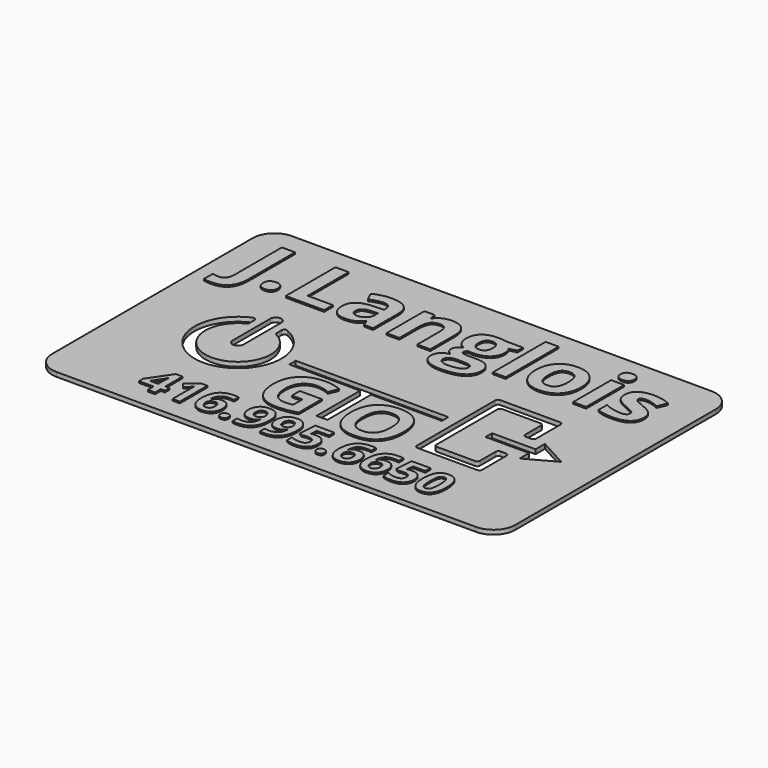
from build123d import *

# Parameters (mm, degrees)
F1_DEPTH       = 0.8
F3_DEPTH       = 0.801
F4_TEXT_SIZE   = 7.0678230889
F5_DEPTH       = 0.3
F6_TEXT_SIZE   = 15.9617374922
F6_TEXT_SIZE_2 = 8.8388333097
F6_TEXT_SIZE_3 = 14.3189125487
F7_DEPTH       = 0.3


# Not quite as in the source:
# - Text() gives the source's letters only with a copy of the font that has no kerning and outlines rounded to 1/6400 em; it was checked with that copy


with BuildPart() as f1:
    # F0 (on Top) → F1 (new body)
    with BuildSketch(Plane.XY):
        with BuildLine():
            ThreePointArc((42.4102088809, 23.1660448015), (41.2386360056, 25.9944719262), (38.4102088809, 27.1660448015))
            Line((38.4102088809, 27.1660448015), (-38.5897911191, 27.1660448015))
            ThreePointArc((-38.5897911191, 27.1660448015), (-41.4182182438, 25.9944719262), (-42.5897911191, 23.1660448015))
            Line((-42.5897911191, 23.1660448015), (-42.5897911191, -22.8339551985))
            ThreePointArc((-42.5897911191, -22.8339551985), (-41.4182182438, -25.6623823233), (-38.5897911191, -26.8339551985))
            Line((-38.5897911191, -26.8339551985), (38.4102088809, -26.8339551985))
            ThreePointArc((38.4102088809, -26.8339551985), (41.2386360056, -25.6623823233), (42.4102088809, -22.8339551985))
            Line((42.4102088809, -22.8339551985), (42.4102088809, 23.1660448015))
        make_face()
    extrude(amount=F1_DEPTH)

    # F2 (on face) → F3 (cut, through all)
    with BuildSketch(Plane.XY.offset(0.8)):
        with BuildLine():
            ThreePointArc((-21.2221585948, 1.8853944422), (-23.991389364, -9.4373267554), (-26.7606201332, 1.8853944422))
            ThreePointArc((-26.7606201332, 1.8853944422), (-26.5639641569, 2.0695172811), (-26.491389364, 2.328954542))
            Line((-26.491389364, 2.328954542), (-26.491389364, 3.4365367871))
            ThreePointArc((-26.491389364, 3.4365367871), (-26.7175280853, 3.8548668003), (-27.191389364, 3.8947943566))
            ThreePointArc((-27.191389364, 3.8947943566), (-23.991389364, -11.4373267554), (-20.791389364, 3.8947943566))
            ThreePointArc((-20.791389364, 3.8947943566), (-21.2652506428, 3.8548668003), (-21.491389364, 3.4365367871))
            Line((-21.491389364, 3.4365367871), (-21.491389364, 2.328954542))
            ThreePointArc((-21.491389364, 2.328954542), (-21.4188145711, 2.0695172811), (-21.2221585948, 1.8853944422))
        make_face()
        with BuildLine():
            ThreePointArc((18.008610636, 3.5626732446), (18.1550572454, 3.9162266352), (18.508610636, 4.0626732446))
            Line((18.508610636, 4.0626732446), (25.508610636, 4.0626732446))
            ThreePointArc((25.508610636, 4.0626732446), (25.8621640266, 3.9162266352), (26.008610636, 3.5626732446))
            Line((26.008610636, 3.5626732446), (26.008610636, -0.0391275138))
            ThreePointArc((26.008610636, -0.0391275138), (26.1550572454, -0.3926809044), (26.508610636, -0.5391275138))
            Line((26.508610636, -0.5391275138), (27.508610636, -0.5391275138))
            ThreePointArc((27.508610636, -0.5391275138), (27.8621640266, -0.3926809044), (28.008610636, -0.0391275138))
            Line((28.008610636, -0.0391275138), (28.008610636, 5.5626732446))
            ThreePointArc((28.008610636, 5.5626732446), (27.8621640266, 5.9162266352), (27.508610636, 6.0626732446))
            Line((27.508610636, 6.0626732446), (16.508610636, 6.0626732446))
            ThreePointArc((16.508610636, 6.0626732446), (16.1550572454, 5.9162266352), (16.008610636, 5.5626732446))
            Line((16.008610636, 5.5626732446), (16.008610636, -12.4373267554))
            ThreePointArc((16.008610636, -12.4373267554), (16.1550572454, -12.790880146), (16.508610636, -12.9373267554))
            Line((16.508610636, -12.9373267554), (27.508610636, -12.9373267554))
            ThreePointArc((27.508610636, -12.9373267554), (27.8621640266, -12.790880146), (28.008610636, -12.4373267554))
            Line((28.008610636, -12.4373267554), (28.008610636, -6.835525997))
            ThreePointArc((28.008610636, -6.835525997), (27.8621640266, -6.4819726064), (27.508610636, -6.335525997))
            Line((27.508610636, -6.335525997), (26.508610636, -6.335525997))
            ThreePointArc((26.508610636, -6.335525997), (26.1550572454, -6.4819726064), (26.008610636, -6.835525997))
            Line((26.008610636, -6.835525997), (26.008610636, -10.4373267554))
            ThreePointArc((26.008610636, -10.4373267554), (25.8621640266, -10.790880146), (25.508610636, -10.9373267554))
            Line((25.508610636, -10.9373267554), (18.508610636, -10.9373267554))
            ThreePointArc((18.508610636, -10.9373267554), (18.1550572454, -10.790880146), (18.008610636, -10.4373267554))
            Line((18.008610636, -10.4373267554), (18.008610636, 3.5626732446))
        make_face()
        with BuildLine():
            ThreePointArc((-24.991389364, -3.4373267554), (-23.991389364, -4.4373267554), (-22.991389364, -3.4373267554))
            Line((-22.991389364, -3.4373267554), (-22.991389364, 5.2381165931))
            ThreePointArc((-22.991389364, 5.2381165931), (-23.991389364, 6.2381165931), (-24.991389364, 5.2381165931))
            Line((-24.991389364, 5.2381165931), (-24.991389364, -3.4373267554))
        make_face()
        with BuildLine():
            ThreePointArc((-14.0195540264, -2.6873267554), (-13.991389364, -3.4373267554), (-14.0195540264, -4.1873267554))
            Line((-14.0195540264, -4.1873267554), (-0.991389364, -4.1873267554))
            Line((-0.991389364, -4.1873267554), (-0.991389364, -14.1873267554))
            Line((-0.991389364, -14.1873267554), (1.008610636, -14.1873267554))
            Line((1.008610636, -14.1873267554), (1.008610636, -4.1873267554))
            Line((1.008610636, -4.1873267554), (14.008610636, -4.1873267554))
            Line((14.008610636, -4.1873267554), (14.008610636, -2.6873267554))
            Line((14.008610636, -2.6873267554), (-14.0195540264, -2.6873267554))
        make_face()
        Polygon((30.008610636, -2.6873267554), (22.008610636, -2.6873267554), (22.008610636, -4.1873267554), (30.008610636, -4.1873267554), (30.0109457225, -6.335525997), (35.3433839977, -3.4373267554), (30.0109457225, -0.5391275138), align=None)
    extrude(amount=-F3_DEPTH, mode=Mode.SUBTRACT)

    # F4 (on face) → F5 (cut)
    with BuildSketch(Plane(origin=(0, 0, 0), x_dir=(1, 0, 0), z_dir=(0, 0, -1))):
        with Locations((-41, -15.4066556562)):
            Text('www.GrayToqueOps.ca', F4_TEXT_SIZE, font='Open Sans', font_style=FontStyle.BOLD, text_align=(TextAlign.LEFT, TextAlign.BOTTOM))
    extrude(amount=-F5_DEPTH, mode=Mode.SUBTRACT)

    # F6 (on face) → F7 (join)
    with BuildSketch(Plane.XY.offset(0.8)):
        with Locations((-38.5897911191, 11.6735938071)):
            Text('J.Langlois', F6_TEXT_SIZE, font='Open Sans', font_style=FontStyle.BOLD, text_align=(TextAlign.LEFT, TextAlign.BOTTOM))
        with Locations((-27.3866634816, -23.4203394502)):
            Text('416.995.6650', F6_TEXT_SIZE_2, font='Open Sans', font_style=FontStyle.BOLD, text_align=(TextAlign.LEFT, TextAlign.BOTTOM))
        with Locations((-12.4865729595, -15.859794803)):
            Text('G', F6_TEXT_SIZE_3, font='Open Sans', font_style=FontStyle.BOLD, text_align=(TextAlign.LEFT, TextAlign.BOTTOM))
        with Locations((1.676385873, -15.859794803)):
            Text('O', F6_TEXT_SIZE_3, font='Open Sans', font_style=FontStyle.BOLD, text_align=(TextAlign.LEFT, TextAlign.BOTTOM))
    extrude(amount=F7_DEPTH)


solid = f1.part
